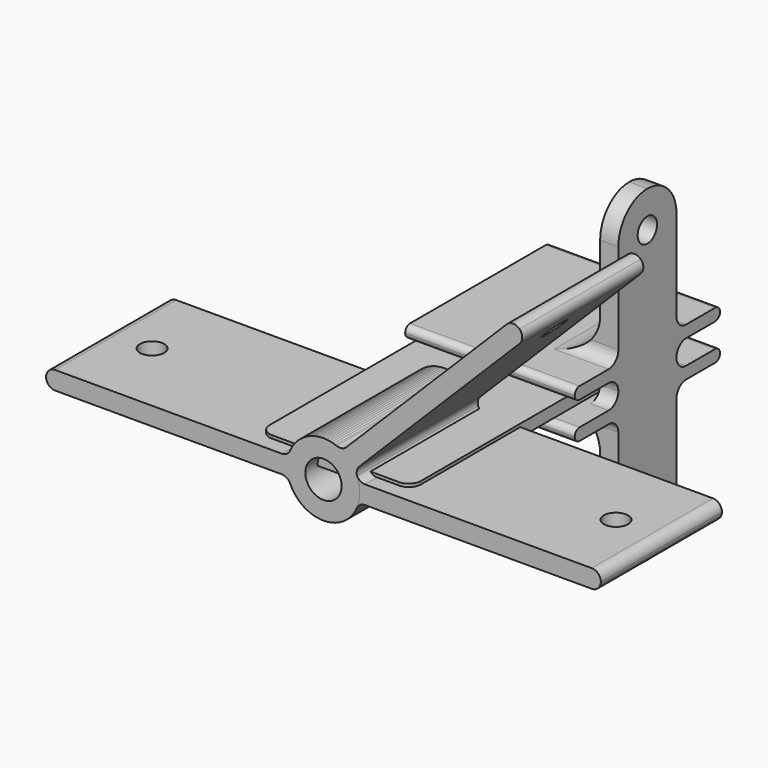
from build123d import *

# Parameters (mm, degrees)
F0_R      = 3
F1_DEPTH  = 25
F2_R      = 1.49999
F3_R      = 3
F4_DEPTH  = 25
F5_R      = 1.49999
F7_R      = 2
F8_DEPTH  = 3
F6_R      = 2
F9_R      = 2
F10_DEPTH = 3
F11_W     = 25
F11_H     = 45
F11_R     = 2
F12_DEPTH = 2
F13_W     = 12
F13_H     = 23
F13_R     = 2
F13_W_2   = 9
F13_H_2   = 2
F13_W_3   = 6
F14_DEPTH = 3
F15_DEPTH = 25
F16_R     = 0.99999
F17_R     = 5.99999
F18_R     = 1.99999
F19_R     = 2


# Not quite as in the source:
# - a fillet or chamfer is up to 0.001 mm smaller than in the source, because OpenCascade refuses the exact size


with BuildPart() as f1:
    # F0 (on Front) → F1 (new body)
    with BuildSketch(Plane.XZ):
        with BuildLine():
            ThreePointArc((-5.8094750193, -1.5), (-6, 0), (-5.8094750193, 1.5))
            Line((-5.8094750193, 1.5), (-45.8094750193, 1.5))
            Line((-45.8094750193, 1.5), (-45.8094750193, -1.5))
            Line((-45.8094750193, -1.5), (-5.8094750193, -1.5))
        make_face()
        with BuildLine():
            ThreePointArc((5.8094750193, -1.5), (5.9521781776, -0.7560257549), (6, 0))
            ThreePointArc((6, 0), (5.9521781776, 0.7560257549), (5.8094750193, 1.5))
            ThreePointArc((5.8094750193, 1.5), (0, 6), (-5.8094750193, 1.5))
            ThreePointArc((-5.8094750193, 1.5), (-6, 0), (-5.8094750193, -1.5))
            ThreePointArc((-5.8094750193, -1.5), (0, -6), (5.8094750193, -1.5))
        make_face()
        Circle(F0_R, mode=Mode.SUBTRACT)
        with BuildLine():
            ThreePointArc((5.8094750193, 1.5), (5.9521781776, 0.7560257549), (6, 0))
            ThreePointArc((6, 0), (5.9521781776, -0.7560257549), (5.8094750193, -1.5))
            Line((5.8094750193, -1.5), (45.8094750193, -1.5))
            Line((45.8094750193, -1.5), (45.8094750193, 1.5))
            Line((45.8094750193, 1.5), (5.8094750193, 1.5))
        make_face()
    extrude(amount=F1_DEPTH)

    # F2 (radius 1.5 in the source; OpenCascade refuses exactly that, so slightly less here)
    f2_edges = [f1.edges().sort_by_distance(p)[0] for p in [
        (-45.809475, -12.5, 1.5),
        (-45.809475, -12.5, -1.5),
        (45.809475, -12.5, 1.5),
        (45.809475, -12.5, -1.5),
        (-5.809475, -12.5, 1.5),
        (5.809475, -12.5, 1.5),
        (-5.809475, -12.5, -1.5),
        (5.809475, -12.5, -1.5),
    ]]
    fillet(f2_edges, radius=F2_R)


with BuildPart() as f4:
    # F3 (on Front) → F4 (new body)
    with BuildSketch(Plane.XZ):
        with BuildLine():
            Line((-45.8094750193, -1.5), (-5.8094750193, -1.5))
            ThreePointArc((-5.8094750193, -1.5), (-6, 0), (-5.8094750193, 1.5))
            Line((-5.8094750193, 1.5), (-45.8094750193, 1.5))
            Line((-45.8094750193, 1.5), (-45.8094750193, -1.5))
        make_face()
        with BuildLine():
            ThreePointArc((-5.8094750193, -1.5), (0.7560257549, -5.9521781776), (6, 0))
            ThreePointArc((6, 0), (5.788414123, 1.5793232541), (5.1685793531, 3.0472590095))
            ThreePointArc((5.1685793531, 3.0472590095), (4.2426406871, 4.2426406871), (3.0472590095, 5.1685793531))
            ThreePointArc((3.0472590095, 5.1685793531), (-2.2961005942, 5.5432771951), (-5.8094750193, 1.5))
            ThreePointArc((-5.8094750193, 1.5), (-6, 0), (-5.8094750193, -1.5))
        make_face()
        Circle(F3_R, mode=Mode.SUBTRACT)
        with BuildLine():
            ThreePointArc((3.0472590095, 5.1685793531), (4.2426406871, 4.2426406871), (5.1685793531, 3.0472590095))
            Line((5.1685793531, 3.0472590095), (33.4528506005, 31.331530257))
            Line((33.4528506005, 31.331530257), (31.331530257, 33.4528506005))
            Line((31.331530257, 33.4528506005), (3.0472590095, 5.1685793531))
        make_face()
    extrude(amount=F4_DEPTH)

    # F5 (radius 1.5 in the source; OpenCascade refuses exactly that, so slightly less here)
    f5_edges = [f4.edges().sort_by_distance(p)[0] for p in [
        (-45.809475, -12.5, 1.5),
        (-5.809475, -12.5, 1.5),
        (3.047259, -12.5, 5.168579),
        (31.33153, -12.5, 33.452851),
        (33.452851, -12.5, 31.33153),
        (-45.809475, -12.5, -1.5),
        (-5.809475, -12.5, -1.5),
        (5.168579, -12.5, 3.047259),
    ]]
    fillet(f5_edges, radius=F5_R)

    # F7 (on face) → F8 (cut, through all)
    with BuildSketch(Plane(origin=(1.0606601718, 0, -1.0606601718), x_dir=(0, 1, 0), z_dir=(0.7071067812, 0, -0.7071067812))):
        with Locations((-12.5, 38.3094750193)):
            Circle(F7_R)
    extrude(amount=-F8_DEPTH, mode=Mode.SUBTRACT)


with BuildPart() as f10_tool:
    # F6 (on face) + F9 (on face) → F10 (new body, through all)
    with BuildSketch(Plane(origin=(0, 0, -1.5), x_dir=(1, 0, 0), z_dir=(0, 0, -1))):
        with Locations((-38.3094750193, 12.5)):
            Circle(F6_R)
    with BuildSketch(Plane(origin=(0, 0, -1.5), x_dir=(1, 0, 0), z_dir=(0, 0, -1))):
        with Locations((38.3094750193, 12.5)):
            Circle(F9_R)
    extrude(amount=-F10_DEPTH)


with BuildPart() as f1_1:
    add(f1.part)

    # F10: cut by f10_tool
    add(f10_tool.part, mode=Mode.SUBTRACT)


with BuildPart() as f4_1:
    add(f4.part)

    # F10: cut by f10_tool
    add(f10_tool.part, mode=Mode.SUBTRACT)


with BuildPart() as f12:
    # F11 (on Top) → F12 (new body)
    with BuildSketch(Plane.XY):
        Rectangle(F11_W, F11_H)
        with Locations((0, 16.5)):
            Circle(F11_R, mode=Mode.SUBTRACT)
    extrude(amount=F12_DEPTH)

    # F19
    f19_edges = [f12.edges().sort_by_distance(p)[0] for p in [
        (-12.5, -22.5, 1),
        (12.5, -22.5, 1),
        (12.5, 22.5, 1),
        (-12.5, 22.5, 1),
    ]]
    fillet(f19_edges, radius=F19_R)


with BuildPart() as f14:
    # F13 (on face) → F14 (new body)
    with BuildSketch(Plane.YZ.offset(12.5)):
        with Locations((22.5, 16.5)):
            Rectangle(F13_W, F13_H)
        with Locations((22.5, 22)):
            Circle(F13_R, mode=Mode.SUBTRACT)
        with Locations((22.5, -14.5)):
            Rectangle(F13_W, F13_H)
        with Locations((22.5, -20)):
            Circle(F13_R, mode=Mode.SUBTRACT)
        with Locations((33, 4)):
            Rectangle(F13_W_2, F13_H_2)
        with Locations((22.5, 4)):
            Rectangle(F13_W, F13_H_2)
        with Locations((12, 4)):
            Rectangle(F13_W_2, F13_H_2)
        with Locations((12, -2)):
            Rectangle(F13_W_2, F13_H_2)
        with Locations((22.5, -2)):
            Rectangle(F13_W, F13_H_2)
        with Locations((33, -2)):
            Rectangle(F13_W_2, F13_H_2)
        with Locations((19.5, 1)):
            Rectangle(F13_W_3, F13_H_2)
        Polygon((22.5, 2), (22.5, 0), (16.5, 0), (16.5, -1), (28.5, -1), (28.5, 3), (16.5, 3), (16.5, 2), align=None)
    extrude(amount=F14_DEPTH)

    # F13 (on face) → F15 (join, through all)
    with BuildSketch(Plane.YZ.offset(12.5)):
        with Locations((22.5, 4)):
            Rectangle(F13_W, F13_H_2)
        with Locations((12, 4)):
            Rectangle(F13_W_2, F13_H_2)
        with Locations((33, 4)):
            Rectangle(F13_W_2, F13_H_2)
        with Locations((33, -2)):
            Rectangle(F13_W_2, F13_H_2)
        with Locations((22.5, -2)):
            Rectangle(F13_W, F13_H_2)
        with Locations((12, -2)):
            Rectangle(F13_W_2, F13_H_2)
    extrude(amount=-F15_DEPTH)

    # F16 (radius 1 in the source; OpenCascade refuses exactly that, so slightly less here)
    f16_edges = [f14.edges().sort_by_distance(p)[0] for p in [
        (1.5, 7.5, 5),
        (1.5, 7.5, 3),
        (1.5, 37.5, 5),
        (1.5, 37.5, 3),
        (1.5, 37.5, -1),
        (1.5, 37.5, -3),
        (1.5, 7.5, -3),
        (1.5, 7.5, -1),
    ]]
    fillet(f16_edges, radius=F16_R)

    # F17 (radius 6 in the source; OpenCascade refuses exactly that, so slightly less here)
    f17_edges = [f14.edges().sort_by_distance(p)[0] for p in [
        (14, 16.5, -26),
        (14, 28.5, -26),
        (12.5, 22.5, -3),
        (12.5, 22.5, 5),
        (14, 28.5, 28),
        (14, 16.5, 28),
    ]]
    fillet(f17_edges, radius=F17_R)

    # F18 (radius 2 in the source; OpenCascade refuses exactly that, so slightly less here)
    f18_edges = [f14.edges().sort_by_distance(p)[0] for p in [
        (14, 28.5, -3),
        (14, 16.5, -3),
        (14, 28.5, 5),
        (14, 16.5, 5),
        (14, 28.5, 3),
        (14, 28.5, -1),
        (14, 16.5, 3),
        (14, 16.5, -1),
    ]]
    fillet(f18_edges, radius=F18_R)


solid = Compound([f1_1.part, f4_1.part, f12.part, f14.part])
